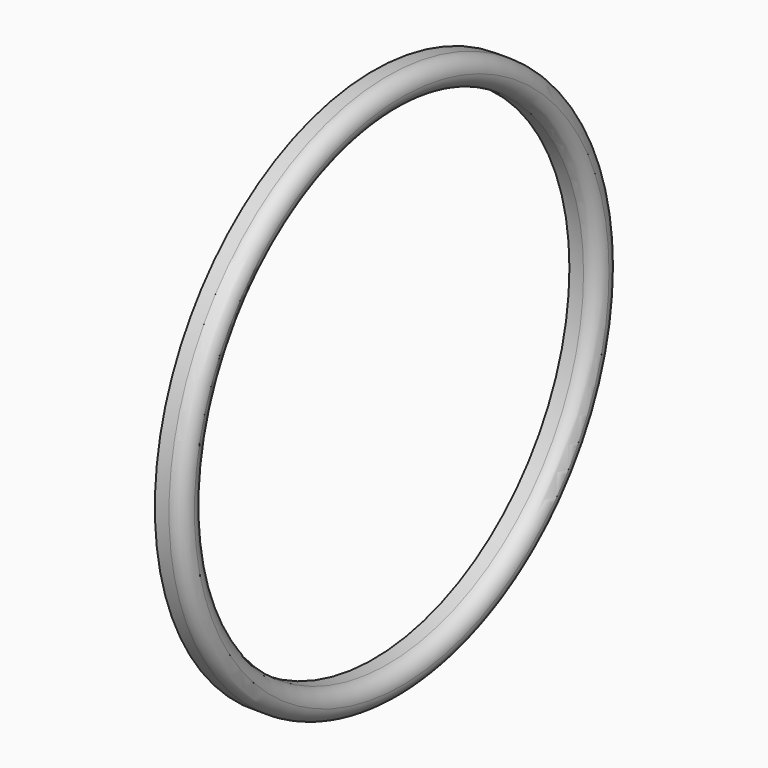
from build123d import *

# Parameters (mm, degrees)
F0_R     = 29
F0_R_2   = 26
F1_DEPTH = 3
F2_R     = 1.49999


# Not quite as in the source:
# - a fillet or chamfer is up to 0.001 mm smaller than in the source, because OpenCascade refuses the exact size


with BuildPart() as f1:
    # F0 (on Right) → F1 (new body)
    with BuildSketch(Plane.YZ):
        with Locations((-28.0447434634, 32.9113304615)):
            Circle(F0_R)
        with Locations((-28.0447434634, 32.9113304615)):
            Circle(F0_R_2, mode=Mode.SUBTRACT)
    extrude(amount=F1_DEPTH)

    # F2 (radius 1.5 in the source; OpenCascade refuses exactly that, so slightly less here)
    f2_edges = [f1.edges().sort_by_distance(p)[0] for p in [
        (3, -57.044743, 32.91133),
        (3, -54.044743, 32.91133),
    ]]
    fillet(f2_edges, radius=F2_R)


solid = f1.part
